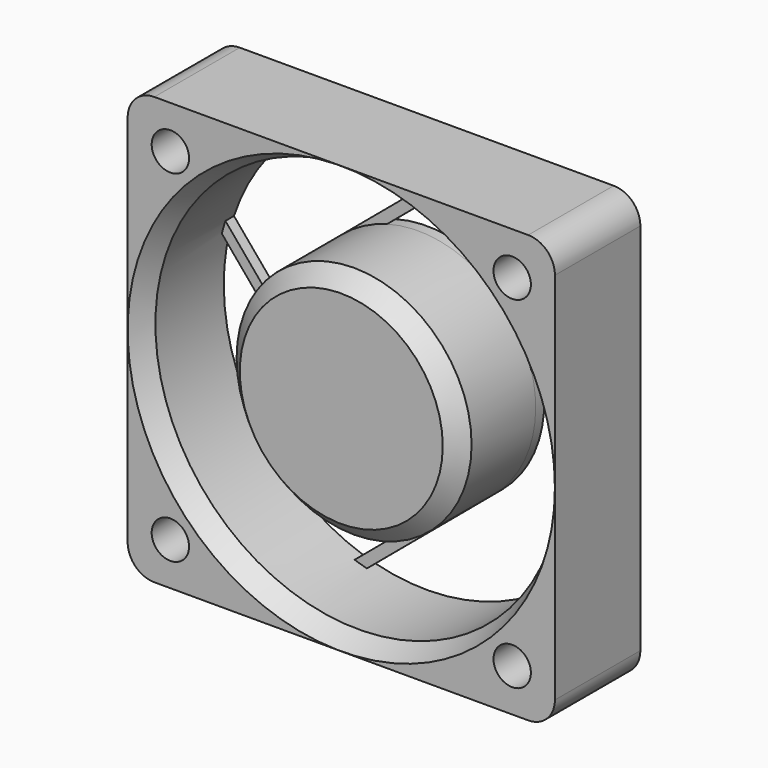
from build123d import *

# Parameters (mm, degrees)
F0_R     = 1.75
F0_R_2   = 19
F1_DEPTH = 10
F3_DEPTH = 1
F4_R     = 11
F5_DEPTH = 9
F7_SIZE2 = 0.99999
F7_SIZE  = 1.99999


# Not quite as in the source:
# - a fillet or chamfer that OpenCascade refuses, or shapes differently, is made with other operations: its cross-section is extruded or revolved along the edge and cut away or added
# - a fillet or chamfer is up to 0.001 mm smaller than in the source, because OpenCascade refuses the exact size


with BuildPart() as f1:
    # F0 (on Front) → F1 (new body)
    with BuildSketch(Plane.XZ):
        with BuildLine():
            Line((-17.5, -20), (17.5, -20))
            ThreePointArc((17.5, -20), (19.267766953, -19.267766953), (20, -17.5))
            Line((20, -17.5), (20, 17.5))
            ThreePointArc((20, 17.5), (19.267766953, 19.267766953), (17.5, 20))
            Line((17.5, 20), (-17.5, 20))
            ThreePointArc((-17.5, 20), (-19.267766953, 19.267766953), (-20, 17.5))
            Line((-20, 17.5), (-20, -17.5))
            ThreePointArc((-20, -17.5), (-19.267766953, -19.267766953), (-17.5, -20))
        make_face()
        with Locations((-16, -16)):
            Circle(F0_R, mode=Mode.SUBTRACT)
        with Locations((16, -16)):
            Circle(F0_R, mode=Mode.SUBTRACT)
        with Locations((-16, 16)):
            Circle(F0_R, mode=Mode.SUBTRACT)
        Circle(F0_R_2, mode=Mode.SUBTRACT)
        with Locations((16, 16)):
            Circle(F0_R, mode=Mode.SUBTRACT)
    extrude(amount=F1_DEPTH)

    # F2 (on Front) → F3 (join)
    with BuildSketch(Plane.XZ):
        with BuildLine():
            Line((5.6323262572, 19.0855630677), (-7.0706637066, 8.4264888743))
            ThreePointArc((-7.0706637066, 8.4264888743), (-10.5017983633, 3.2729544964), (-10.6060673084, -2.9174194506))
            Line((-10.6060673084, -2.9174194506), (-18.3195186246, 6.2751138669))
            Line((-18.3195186246, 6.2751138669), (-19.0855630677, 5.6323262572))
            Line((-19.0855630677, 5.6323262572), (-8.4264888743, -7.0706637066))
            ThreePointArc((-8.4264888743, -7.0706637066), (-3.2729544964, -10.5017983633), (2.9174194506, -10.6060673084))
            Line((2.9174194506, -10.6060673084), (-6.2751138669, -18.3195186246))
            Line((-6.2751138669, -18.3195186246), (-5.6323262572, -19.0855630677))
            Line((-5.6323262572, -19.0855630677), (7.0706637066, -8.4264888743))
            ThreePointArc((7.0706637066, -8.4264888743), (10.5017983633, -3.2729544964), (10.6060673084, 2.9174194506))
            Line((10.6060673084, 2.9174194506), (18.3195186246, -6.2751138669))
            Line((18.3195186246, -6.2751138669), (19.0855630677, -5.6323262572))
            Line((19.0855630677, -5.6323262572), (8.4264888743, 7.0706637066))
            ThreePointArc((8.4264888743, 7.0706637066), (3.2729544964, 10.5017983633), (-2.9174194506, 10.6060673084))
            Line((-2.9174194506, 10.6060673084), (6.2751138669, 18.3195186246))
            Line((6.2751138669, 18.3195186246), (5.6323262572, 19.0855630677))
        make_face()
    extrude(amount=F3_DEPTH)

    # F4 (on face) → F5 (join)
    with BuildSketch(Plane.XZ.offset(1)):
        Circle(F4_R)
    extrude(amount=F5_DEPTH)

    # F6: chamfer of 1.5 on 1 edges, made by hand

    # F6_s1 → F6_t2 (revolve, cut)
    with BuildSketch(Plane.XY):
        Polygon((11, -8.5), (9.5, -10), (11, -10), align=None)
    revolve(axis=Axis((0, -10, 0), (0, -1, 0)), mode=Mode.SUBTRACT)

    # F7 (size 2 and 1 in the source; OpenCascade refuses exactly that, so slightly less here)
    f7_edges = [f1.edges().sort_by_distance(p)[0] for p in [
        (-19, -10, 0),
    ]]
    f7_side = f1.faces().sort_by_distance((-19, -5, 0))[0]
    chamfer(f7_edges, length=F7_SIZE, length2=F7_SIZE2, reference=f7_side)


solid = f1.part
